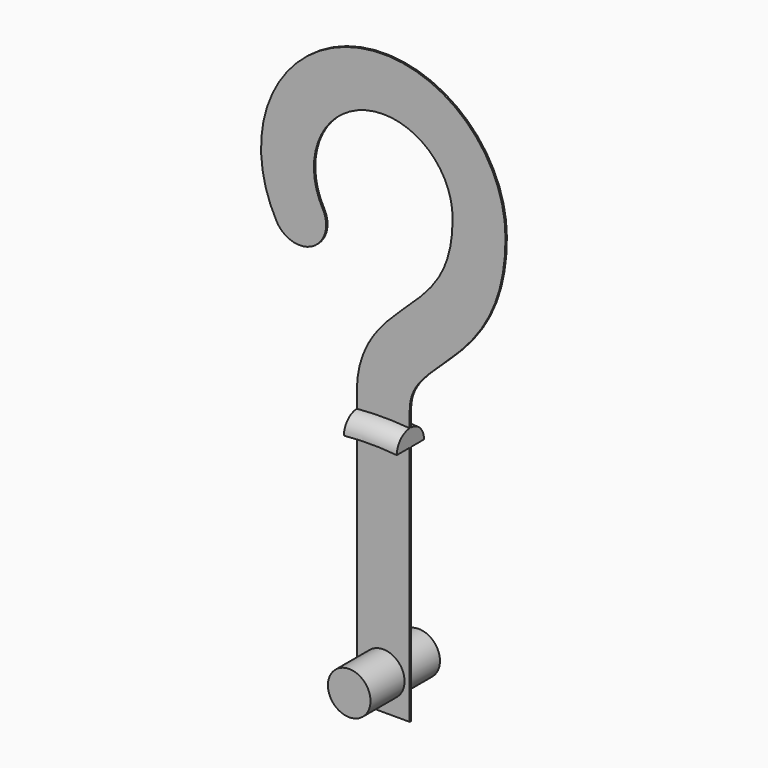
from build123d import *

# Parameters (mm, degrees)
F1_R        = 3.175
F2_DEPTH    = 0.127
F3_DEPTH    = 6.477
F4_DEPTH    = 2.54
F5_T2_ANGLE = 26.9167651383
F6_T2_ANGLE = 26.9167651383


# Not quite as in the source:
# - a fillet or chamfer that OpenCascade refuses, or shapes differently, is made with other operations: its cross-section is extruded or revolved along the edge and cut away or added
# - the dataset's text gives a spline's control points without its knots; the knots are read off the source's solid
# - a feature names something its author has since deleted; it is built from what else it names


with BuildPart() as f2:
    # F1 (on Front) → F2 (new body, symmetric)
    with BuildSketch(Plane.XZ):
        with BuildLine():
            add(Edge.make_bspline(
                [(3.9443914, 49.0440574087), (3.9443914, 49.5051907561), (4.0192504483, 50.3141787289), (4.2927696799, 51.3145496915), (4.7238665835, 52.2424981263), (5.3492657421, 53.1914680624), (6.1938498701, 54.1984330454), (7.6016381276, 55.6371224281), (9.8131344594, 57.6465347772), (12.3123195612, 60.1475954188), (14.2346632912, 62.6261348949), (15.5607778662, 64.7615445573), (16.6924269347, 67.1958901851), (17.8471737016, 70.8493446268), (18.2313183475, 74.0426448984), (18.2313183475, 76.3900893487)],
                knots=[0, 0, 0, 0, 0.0625, 0.125, 0.1875, 0.25, 0.3125, 0.375, 0.5, 0.625, 0.6875, 0.75, 0.8125, 0.875, 1, 1, 1, 1], degree=3))
            ThreePointArc((18.2313183475, 76.3900893487), (-4.6067480226, 94.0297843955), (-15.9032226016, 67.4755798516))
            ThreePointArc((-15.9032226016, 67.4755798516), (-10.5338440854, 65.9635542624), (-9.0218184962, 71.3329327786))
            ThreePointArc((-9.0218184962, 71.3329327786), (-2.6133850704, 86.3969999621), (10.3425355475, 76.3900893487))
            add(Edge.make_bspline(
                [(-3.9443914, 49.0440574087), (-3.9443914, 49.9382927218), (-3.7960172147, 51.6706209873), (-3.1486993579, 54.0540764625), (-2.1566843976, 56.1619218737), (-0.9404093794, 57.9808285198), (0.3915305198, 59.5539381831), (2.2206241488, 61.411766185), (4.4737924881, 63.4540723666), (6.4392720574, 65.4469281755), (7.753810214, 67.1493019234), (8.6042196661, 68.5225825388), (9.3142447745, 70.0500478766), (10.0569804928, 72.3899894099), (10.3425355475, 74.6117631348), (10.3425355475, 76.3900893487)],
                knots=[0, 0, 0, 0, 0.0625, 0.125, 0.1875, 0.25, 0.3125, 0.375, 0.5, 0.625, 0.6875, 0.75, 0.8125, 0.875, 1, 1, 1, 1], degree=3))
            Line((-3.9443914, 49.0440574087), (-3.9444022474, 48.8551537909))
            Line((-3.9444022474, 48.8551537909), (-3.9444022474, 46.7722471395))
            ThreePointArc((-3.9444022474, 46.7722471395), (0, 46.9501537909), (3.9444022474, 46.7722471395))
            Line((3.9444022474, 46.7722471395), (3.9444022474, 48.8551537909))
            Line((3.9444022474, 48.8551537909), (3.9443914, 49.0440574087))
        make_face()
        with BuildLine():
            Line((3.9444022474, 44.2212501729), (3.9444022474, 46.7722471395))
            ThreePointArc((3.9444022474, 46.7722471395), (0, 46.9501537909), (-3.9444022474, 46.7722471395))
            Line((-3.9444022474, 46.7722471395), (-3.9444022474, 44.2212501729))
            ThreePointArc((-3.9444022474, 44.2212501729), (0, 44.4101537909), (3.9444022474, 44.2212501729))
        make_face()
        with BuildLine():
            Line((3.9444022474, 8.2151537909), (3.9444022474, 44.2212501729))
            ThreePointArc((3.9444022474, 44.2212501729), (0, 44.4101537909), (-3.9444022474, 44.2212501729))
            Line((-3.9444022474, 44.2212501729), (-3.9444022474, 8.2151537909))
            Line((-3.9444022474, 8.2151537909), (3.9444022474, 8.2151537909))
        make_face()
        with Locations((0, 13.2951537909)):
            Circle(F1_R, mode=Mode.SUBTRACT)
    extrude(amount=F2_DEPTH, both=True)

    # F1 (on Front) → F3 (join, symmetric)
    with BuildSketch(Plane.XZ):
        with Locations((0, 13.2951537909)):
            Circle(F1_R)
    extrude(amount=F3_DEPTH, both=True)

    # F1 (on Front) → F4 (join, symmetric)
    with BuildSketch(Plane.XZ):
        with BuildLine():
            Line((3.9444022474, 44.2212501729), (3.9444022474, 46.7722471395))
            ThreePointArc((3.9444022474, 46.7722471395), (0, 46.9501537909), (-3.9444022474, 46.7722471395))
            Line((-3.9444022474, 46.7722471395), (-3.9444022474, 44.2212501729))
            ThreePointArc((-3.9444022474, 44.2212501729), (0, 44.4101537909), (3.9444022474, 44.2212501729))
        make_face()
    extrude(amount=F4_DEPTH, both=True)

    # F5: fillet of radius 2.54 on 1 edges, made by hand

    # F5_s1 → F5_t2 (revolve, cut)
    with BuildSketch(Plane(origin=(-0.7096352197, 0, 0.1698232769), x_dir=(0, 1, 0), z_dir=(0.9725392295, 0, -0.2327390106))):
        with BuildLine():
            ThreePointArc((2.54, 44.3272370391), (1.8404048468, 46.0778112307), (0.127, 46.8640600523))
            Line((0.127, 46.8640600523), (2.54, 46.8640600523))
            Line((2.54, 46.8640600523), (2.54, 44.3272370391))
        make_face()
    revolve(axis=Axis((0, 2.54, 3.1351537909), (0, -1, 0)), revolution_arc=F5_T2_ANGLE, mode=Mode.SUBTRACT)

    # F6: fillet of radius 2.54 on 1 edges, made by hand

    # F6_s1 → F6_t2 (revolve, cut)
    with BuildSketch(Plane(origin=(-0.7096352197, 0, 0.1698232769), x_dir=(0, 1, 0), z_dir=(0.9725392295, 0, -0.2327390106))):
        with BuildLine():
            ThreePointArc((-2.54, 44.3272370391), (-1.8404048468, 46.0778112307), (-0.127, 46.8640600523))
            Line((-0.127, 46.8640600523), (-0.12954, 46.9147965125))
            ThreePointArc((-0.12954, 46.9147965125), (-1.3335, 46.9148600523), (-2.54, 46.9148600523))
            Line((-2.54, 46.9148600523), (-2.5908, 46.8640600523))
            Line((-2.5908, 46.8640600523), (-2.5908, 44.3272370391))
            Line((-2.5908, 44.3272370391), (-2.54, 44.3272370391))
        make_face()
    revolve(axis=Axis((0, -2.54, 3.1351537909), (0, -1, 0)), revolution_arc=F6_T2_ANGLE, mode=Mode.SUBTRACT)


solid = f2.part
